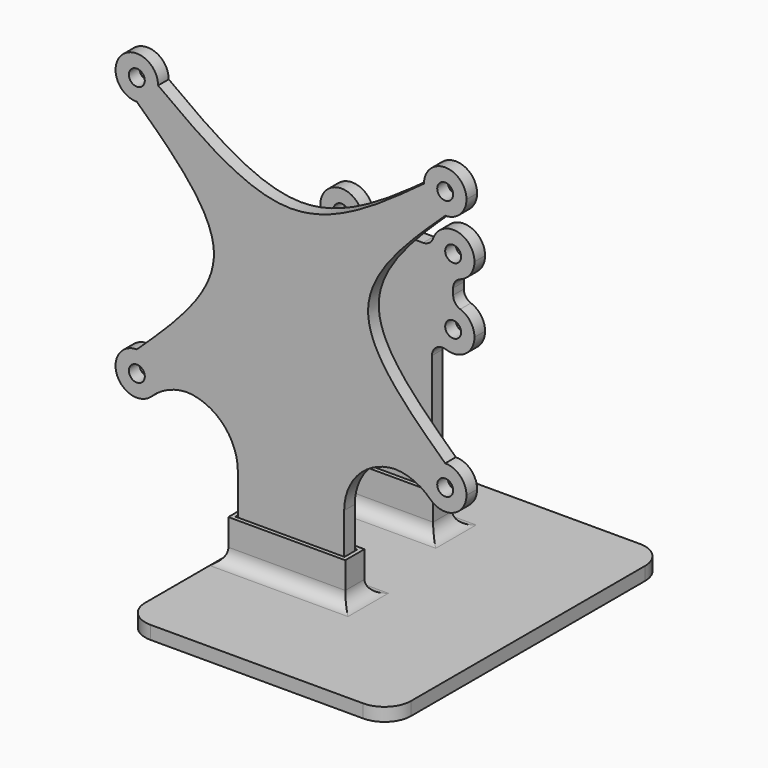
from build123d import *

# Parameters (mm, degrees)
F0_R          = 1.5
F1_DEPTH      = 2.5
F2_T1_DEPTH   = 2.5
F4_R          = 1.5
F4_W          = 13
F4_H          = 30
F5_DEPTH      = 2.5
F6_R          = 2
F7_R          = 2
F9_W          = 25
F9_H          = 65
F9_W_2        = 22
F9_H_2        = 4.5
F9_W_3        = 15
F9_W_4        = 20.5
F9_H_3        = 3
F9_W_5        = 13.5
F10_DEPTH     = 2.5
F11_DEPTH     = 7.5
F12_R         = 5
F13_T1_DEPTH  = 15
F13_T3_DEPTH  = 22
F13_T5_DEPTH  = 4.5
F13_T7_DEPTH  = 4.5
F13_T13_DEPTH = 10.75
F13_T17_DEPTH = 21.25
F13_T24_DEPTH = 21.25
F13_T29_DEPTH = 10.75
F13_T36_DEPTH = 10.75
F13_T40_DEPTH = 28.25
F13_T47_DEPTH = 28.25
F13_T52_DEPTH = 10.2282196187
F13_T59_DEPTH = 21.25
F13_T64_DEPTH = 10.75
F13_T71_DEPTH = 28.25
F13_T76_DEPTH = 10.2282196187
F13_T83_DEPTH = 21.25
F13_T87_DEPTH = 10.75
F13_T94_DEPTH = 28.25
F13_T98_DEPTH = 10.75


# Not quite as in the source:
# - a fillet or chamfer that OpenCascade refuses, or shapes differently, is made with other operations: its cross-section is extruded or revolved along the edge and cut away or added


with BuildPart() as f1:
    # F0 (on Front) → F1 (new body)
    with BuildSketch(Plane.XZ):
        with BuildLine():
            ThreePointArc((-29, 65), (-26.1715728753, 66.1715728753), (-25, 69))
            ThreePointArc((-25, 69), (-31.8284271247, 71.8284271247), (-29, 65))
        make_face()
        with Locations((-29, 69)):
            Circle(F0_R, mode=Mode.SUBTRACT)
        with BuildLine():
            add(Edge.make_bspline(
                [(-25, 69), (-16.6666666667, 62.875), (0, 50.625), (16.6666666667, 62.875), (25, 69)],
                knots=[0, 0, 0, 0, 0.5, 1, 1, 1, 1], degree=3))
            ThreePointArc((-25, 69), (-26.1715728753, 66.1715728753), (-29, 65))
            add(Edge.make_bspline(
                [(-29, 65), (-21.75, 58.1666666667), (-7.25, 44.5), (-21.75, 30.8333333333), (-29, 24)],
                knots=[0, 0, 0, 0, 0.5, 1, 1, 1, 1], degree=3))
            ThreePointArc((-29, 24), (-26.1715728753, 22.8284271247), (-25, 20))
            Line((-25, 20), (-10, 20))
            Line((-10, 20), (-10, 0))
            Line((-10, 0), (10, 0))
            Line((10, 0), (10, 20))
            Line((10, 20), (25, 20))
            ThreePointArc((25, 20), (26.1715728753, 22.8284271247), (29, 24))
            add(Edge.make_bspline(
                [(29, 65), (21.75, 58.1666666667), (7.25, 44.5), (21.75, 30.8333333333), (29, 24)],
                knots=[0, 0, 0, 0, 0.5, 1, 1, 1, 1], degree=3))
            ThreePointArc((29, 65), (26.1715728753, 66.1715728753), (25, 69))
        make_face()
        with BuildLine():
            ThreePointArc((33, 69), (29, 73), (25, 69))
            ThreePointArc((25, 69), (26.1715728753, 66.1715728753), (29, 65))
            ThreePointArc((29, 65), (31.8284271247, 66.1715728753), (33, 69))
        make_face()
        with Locations((29, 69)):
            Circle(F0_R, mode=Mode.SUBTRACT)
        with BuildLine():
            ThreePointArc((-25, 20), (-26.1715728753, 22.8284271247), (-29, 24))
            ThreePointArc((-29, 24), (-31.8284271247, 17.1715728753), (-25, 20))
        make_face()
        with Locations((-29, 20)):
            Circle(F0_R, mode=Mode.SUBTRACT)
        with BuildLine():
            ThreePointArc((33, 20), (31.8284271247, 22.8284271247), (29, 24))
            ThreePointArc((29, 24), (26.1715728753, 22.8284271247), (25, 20))
            ThreePointArc((25, 20), (29, 16), (33, 20))
        make_face()
        with Locations((29, 20)):
            Circle(F0_R, mode=Mode.SUBTRACT)
    extrude(amount=F1_DEPTH)

    # F2: fillet of radius 10 on 4 edges, made by hand

    # F2_s2 → F2_t1 (join)
    with BuildSketch(Plane.XZ):
        with BuildLine():
            ThreePointArc((-26.2005831511, 17.1428571429), (-22.981685759, 19.2582009977), (-19.2020410289, 20))
            Line((-19.2020410289, 20), (-25, 20))
            ThreePointArc((-25, 20), (-25.3123403495, 18.4504302848), (-26.2005831511, 17.1428571429))
        make_face()
        with BuildLine():
            ThreePointArc((19.2020410289, 20), (22.981685759, 19.2582009977), (26.2005831511, 17.1428571429))
            ThreePointArc((26.2005831511, 17.1428571429), (25.3123403495, 18.4504302848), (25, 20))
            Line((25, 20), (19.2020410289, 20))
        make_face()
        with BuildLine():
            ThreePointArc((-20, 20), (-12.9289321881, 17.0710678119), (-10, 10))
            Line((-10, 10), (-10, 20))
            Line((-10, 20), (-20, 20))
        make_face()
        with BuildLine():
            ThreePointArc((10, 10), (12.9289321881, 17.0710678119), (20, 20))
            Line((20, 20), (10, 20))
            Line((10, 20), (10, 10))
        make_face()
    extrude(amount=F2_T1_DEPTH)


with BuildPart() as f5:
    # F4 (on offset) → F5 (new body)
    with BuildSketch(Plane.XZ.offset(-25)):
        with BuildLine():
            ThreePointArc((-10.5, 38.5), (-7.6715728753, 39.6715728753), (-6.5, 42.5))
            ThreePointArc((-6.5, 42.5), (-13.3284271247, 45.3284271247), (-10.5, 38.5))
        make_face()
        with Locations((-10.5, 42.5)):
            Circle(F4_R, mode=Mode.SUBTRACT)
        with BuildLine():
            Line((6.5, 42.5), (-6.5, 42.5))
            ThreePointArc((-6.5, 42.5), (-7.6715728753, 39.6715728753), (-10.5, 38.5))
            Line((-10.5, 38.5), (-10.5, 34))
            ThreePointArc((-10.5, 34), (-7.6715728753, 32.8284271247), (-6.5, 30))
            Line((-6.5, 30), (6.5, 30))
            ThreePointArc((6.5, 30), (7.6715728753, 32.8284271247), (10.5, 34))
            Line((10.5, 34), (10.5, 38.5))
            ThreePointArc((10.5, 38.5), (7.6715728753, 39.6715728753), (6.5, 42.5))
        make_face()
        with BuildLine():
            ThreePointArc((14.5, 42.5), (10.5, 46.5), (6.5, 42.5))
            ThreePointArc((6.5, 42.5), (7.6715728753, 39.6715728753), (10.5, 38.5))
            ThreePointArc((10.5, 38.5), (13.3284271247, 39.6715728753), (14.5, 42.5))
        make_face()
        with Locations((10.5, 42.5)):
            Circle(F4_R, mode=Mode.SUBTRACT)
        with BuildLine():
            ThreePointArc((-6.5, 30), (-7.6715728753, 32.8284271247), (-10.5, 34))
            ThreePointArc((-10.5, 34), (-13.3284271247, 27.1715728753), (-6.5, 30))
        make_face()
        with Locations((-10.5, 30)):
            Circle(F4_R, mode=Mode.SUBTRACT)
        with Locations((0, 15)):
            Rectangle(F4_W, F4_H)
        with BuildLine():
            ThreePointArc((14.5, 30), (13.3284271247, 32.8284271247), (10.5, 34))
            ThreePointArc((10.5, 34), (7.6715728753, 32.8284271247), (6.5, 30))
            ThreePointArc((6.5, 30), (10.5, 26), (14.5, 30))
        make_face()
        with Locations((10.5, 30)):
            Circle(F4_R, mode=Mode.SUBTRACT)
    extrude(amount=F5_DEPTH)

    # F6
    f6_edges = [f5.edges().sort_by_distance(p)[0] for p in [
        (-6.5, 23.75, 42.5),
        (6.5, 23.75, 42.5),
        (10.5, 23.75, 38.5),
        (-10.5, 23.75, 38.5),
        (-10.5, 23.75, 34),
        (10.5, 23.75, 34),
    ]]
    fillet(f6_edges, radius=F6_R)

    # F7
    f7_edges = [f5.edges().sort_by_distance(p)[0] for p in [
        (-6.5, 23.75, 30),
        (6.5, 23.75, 30),
    ]]
    fillet(f7_edges, radius=F7_R)


with BuildPart() as f10:
    # F9 (on offset) → F10 (new body)
    with BuildSketch(Plane.XY.offset(-5)):
        with Locations((0, 6.3541418326)):
            Rectangle(F9_W, F9_H)
        with Locations((0, -1.238761819)):
            Rectangle(F9_W_2, F9_H_2, mode=Mode.SUBTRACT)
        with Locations((0, 23.7820465118)):
            Rectangle(F9_W_3, F9_H_2, mode=Mode.SUBTRACT)
        with Locations((25, 6.3541418326)):
            Rectangle(F9_W, F9_H)
        with Locations((0, -1.238761819)):
            Rectangle(F9_W_2, F9_H_2)
        with Locations((0, -1.238761819)):
            Rectangle(F9_W_4, F9_H_3, mode=Mode.SUBTRACT)
        with Locations((0, 23.7820465118)):
            Rectangle(F9_W_3, F9_H_2)
        with Locations((0, 23.7820465118)):
            Rectangle(F9_W_5, F9_H_3, mode=Mode.SUBTRACT)
        with Locations((0, -1.238761819)):
            Rectangle(F9_W_4, F9_H_3)
        with Locations((0, 23.7820465118)):
            Rectangle(F9_W_5, F9_H_3)
    extrude(amount=-F10_DEPTH)

    # F9 (on offset) → F11 (join)
    with BuildSketch(Plane.XY.offset(-5)):
        with Locations((0, 23.7820465118)):
            Rectangle(F9_W_3, F9_H_2)
        with Locations((0, 23.7820465118)):
            Rectangle(F9_W_5, F9_H_3, mode=Mode.SUBTRACT)
        with Locations((0, -1.238761819)):
            Rectangle(F9_W_2, F9_H_2)
        with Locations((0, -1.238761819)):
            Rectangle(F9_W_4, F9_H_3, mode=Mode.SUBTRACT)
    extrude(amount=F11_DEPTH)

    # F12
    f12_edges = [f10.edges().sort_by_distance(p)[0] for p in [
        (-12.5, 38.854142, -6.25),
        (-12.5, -26.145858, -6.25),
        (37.5, -26.145858, -6.25),
        (37.5, 38.854142, -6.25),
    ]]
    fillet(f12_edges, radius=F12_R)

    # F13: fillet of radius 2.5 on 8 edges, made by hand

    # F13_s2 → F13_t1 (join)
    with BuildSketch(Plane.YZ.offset(-7.5)):
        with BuildLine():
            ThreePointArc((28.5320465118, -5), (26.7642795588, -4.267766953), (26.0320465118, -2.5))
            Line((26.0320465118, -2.5), (26.0320465118, -5))
            Line((26.0320465118, -5), (28.5320465118, -5))
        make_face()
        with BuildLine():
            ThreePointArc((19.0320465118, -5), (20.7998134647, -4.267766953), (21.5320465118, -2.5))
            Line((21.5320465118, -2.5), (21.5320465118, -5))
            Line((21.5320465118, -5), (19.0320465118, -5))
        make_face()
    extrude(amount=F13_T1_DEPTH)

    # F13_s4 → F13_t3 (join)
    with BuildSketch(Plane.YZ.offset(-11)):
        with BuildLine():
            ThreePointArc((3.511238181, -5), (1.7434712281, -4.267766953), (1.011238181, -2.5))
            Line((1.011238181, -2.5), (1.011238181, -5))
            Line((1.011238181, -5), (3.511238181, -5))
        make_face()
        with BuildLine():
            ThreePointArc((-5.988761819, -5), (-4.220994866, -4.267766953), (-3.488761819, -2.5))
            Line((-3.488761819, -2.5), (-3.488761819, -5))
            Line((-3.488761819, -5), (-5.988761819, -5))
        make_face()
    extrude(amount=F13_T3_DEPTH)

    # F13_s6 → F13_t5 (join)
    with BuildSketch(Plane.XZ.offset(-26.0320465118)):
        with BuildLine():
            ThreePointArc((-10, -5), (-8.232233047, -4.267766953), (-7.5, -2.5))
            Line((-7.5, -2.5), (-7.5, -5))
            Line((-7.5, -5), (-10, -5))
        make_face()
        with BuildLine():
            ThreePointArc((10, -5), (8.232233047, -4.267766953), (7.5, -2.5))
            Line((7.5, -2.5), (7.5, -5))
            Line((7.5, -5), (10, -5))
        make_face()
    extrude(amount=F13_T5_DEPTH)

    # F13_s8 → F13_t7 (join)
    with BuildSketch(Plane.XZ.offset(-1.011238181)):
        with BuildLine():
            ThreePointArc((-12.5, -5), (-11.4083499337, -4.0780185463), (-11, -2.7087121525))
            Line((-11, -2.7087121525), (-11, -5))
            Line((-11, -5), (-12.5, -5))
        make_face()
        with BuildLine():
            ThreePointArc((13.5, -5), (11.732233047, -4.267766953), (11, -2.5))
            Line((11, -2.5), (11, -5))
            Line((11, -5), (13.5, -5))
        make_face()
    extrude(amount=F13_T7_DEPTH)


with BuildPart() as f13_tool11:
    # F13_s12 → F13_t13 (new body)
    with BuildSketch(Plane.XZ.offset(-21.5320465118)):
        with BuildLine():
            ThreePointArc((10, -5), (8.232233047, -4.267766953), (7.5, -2.5))
            Line((7.5, -2.5), (7.5, -5))
            Line((7.5, -5), (10, -5))
        make_face()
    extrude(amount=-F13_T13_DEPTH)

    split(bisect_by=Plane.XZ.offset(-26.0320465118), keep=Keep.BOTTOM)


with BuildPart() as f13_tool15:
    # F13_s16 → F13_t17 (new body)
    with BuildSketch(Plane.YZ.offset(13.75)):
        with BuildLine():
            ThreePointArc((28.5320465118, -5), (26.7642795588, -4.267766953), (26.0320465118, -2.5))
            Line((26.0320465118, -2.5), (26.0320465118, -5))
            Line((26.0320465118, -5), (28.5320465118, -5))
        make_face()
    extrude(amount=-F13_T17_DEPTH)

    split(bisect_by=Plane.YZ.offset(7.5), keep=Keep.TOP)


with BuildPart() as f13_tool11_1:
    add(f13_tool11.part)

    # F13_t19: intersect F13_tool15
    add(f13_tool15.part, mode=Mode.INTERSECT)


with BuildPart() as f10_1:
    add(f10.part)

    # F13_t9: union F13_tool11
    add(f13_tool11_1.part)


with BuildPart() as f13_tool22:
    # F13_s23 → F13_t24 (new body)
    with BuildSketch(Plane.YZ.offset(7.5)):
        with BuildLine():
            ThreePointArc((28.5320465118, -5), (26.7642795588, -4.267766953), (26.0320465118, -2.5))
            Line((26.0320465118, -2.5), (26.0320465118, -5))
            Line((26.0320465118, -5), (28.5320465118, -5))
        make_face()
    extrude(amount=-F13_T24_DEPTH)

    split(bisect_by=Plane.YZ.offset(-12.5), keep=Keep.TOP)

    split(bisect_by=Plane.YZ.offset(-7.5), keep=Keep.BOTTOM)


with BuildPart() as f13_tool27:
    # F13_s28 → F13_t29 (new body)
    with BuildSketch(Plane.XZ.offset(-32.2820465118)):
        with BuildLine():
            ThreePointArc((-10, -5), (-8.232233047, -4.267766953), (-7.5, -2.5))
            Line((-7.5, -2.5), (-7.5, -5))
            Line((-7.5, -5), (-10, -5))
        make_face()
    extrude(amount=F13_T29_DEPTH)

    split(bisect_by=Plane.XZ.offset(-26.0320465118), keep=Keep.BOTTOM)


with BuildPart() as f13_tool22_1:
    add(f13_tool22.part)

    # F13_t31: intersect F13_tool27
    add(f13_tool27.part, mode=Mode.INTERSECT)


with BuildPart() as f10_2:
    add(f10_1.part)

    # F13_t20: union F13_tool22
    add(f13_tool22_1.part)


with BuildPart() as f13_tool34:
    # F13_s35 → F13_t36 (new body)
    with BuildSketch(Plane.XZ.offset(3.488761819)):
        with BuildLine():
            ThreePointArc((13.5, -5), (11.732233047, -4.267766953), (11, -2.5))
            Line((11, -2.5), (11, -5))
            Line((11, -5), (13.5, -5))
        make_face()
    extrude(amount=-F13_T36_DEPTH)

    split(bisect_by=Plane.XZ.offset(-1.011238181), keep=Keep.BOTTOM)


with BuildPart() as f13_tool38:
    # F13_s39 → F13_t40 (new body)
    with BuildSketch(Plane.YZ.offset(17.25)):
        with BuildLine():
            ThreePointArc((3.511238181, -5), (1.7434712281, -4.267766953), (1.011238181, -2.5))
            Line((1.011238181, -2.5), (1.011238181, -5))
            Line((1.011238181, -5), (3.511238181, -5))
        make_face()
    extrude(amount=-F13_T40_DEPTH)

    split(bisect_by=Plane.YZ.offset(11), keep=Keep.TOP)


with BuildPart() as f13_tool34_1:
    add(f13_tool34.part)

    # F13_t42: intersect F13_tool38
    add(f13_tool38.part, mode=Mode.INTERSECT)


with BuildPart() as f10_3:
    add(f10_2.part)

    # F13_t32: union F13_tool34
    add(f13_tool34_1.part)


with BuildPart() as f13_tool45:
    # F13_s46 → F13_t47 (new body)
    with BuildSketch(Plane.YZ.offset(11)):
        with BuildLine():
            ThreePointArc((3.511238181, -5), (1.7434712281, -4.267766953), (1.011238181, -2.5))
            Line((1.011238181, -2.5), (1.011238181, -5))
            Line((1.011238181, -5), (3.511238181, -5))
        make_face()
    extrude(amount=-F13_T47_DEPTH)

    split(bisect_by=Plane.YZ.offset(-12.5), keep=Keep.TOP)

    split(bisect_by=Plane.YZ.offset(-11), keep=Keep.BOTTOM)


with BuildPart() as f13_tool50:
    # F13_s51 → F13_t52 (new body)
    with BuildSketch(Plane.XZ.offset(-6.7394577997)):
        with BuildLine():
            ThreePointArc((-12.5, -5), (-11.4083499337, -4.0780185463), (-11, -2.7087121525))
            Line((-11, -2.7087121525), (-11, -5))
            Line((-11, -5), (-12.5, -5))
        make_face()
    extrude(amount=F13_T52_DEPTH)

    split(bisect_by=Plane.XZ.offset(-1.011238181), keep=Keep.BOTTOM)


with BuildPart() as f13_tool45_1:
    add(f13_tool45.part)

    # F13_t54: intersect F13_tool50
    add(f13_tool50.part, mode=Mode.INTERSECT)


with BuildPart() as f10_4:
    add(f10_3.part)

    # F13_t43: union F13_tool45
    add(f13_tool45_1.part)


with BuildPart() as f13_tool57:
    # F13_s58 → F13_t59 (new body)
    with BuildSketch(Plane.YZ.offset(-13.75)):
        with BuildLine():
            ThreePointArc((19.0320465118, -5), (20.7998134647, -4.267766953), (21.5320465118, -2.5))
            Line((21.5320465118, -2.5), (21.5320465118, -5))
            Line((21.5320465118, -5), (19.0320465118, -5))
        make_face()
    extrude(amount=F13_T59_DEPTH)

    split(bisect_by=Plane.YZ.offset(-12.5), keep=Keep.TOP)

    split(bisect_by=Plane.YZ.offset(-7.5), keep=Keep.BOTTOM)


with BuildPart() as f13_tool62:
    # F13_s63 → F13_t64 (new body)
    with BuildSketch(Plane.XZ.offset(-26.0320465118)):
        with BuildLine():
            ThreePointArc((-10, -5), (-8.232233047, -4.267766953), (-7.5, -2.5))
            Line((-7.5, -2.5), (-7.5, -5))
            Line((-7.5, -5), (-10, -5))
        make_face()
    extrude(amount=F13_T64_DEPTH)

    split(bisect_by=Plane.XZ.offset(-21.5320465118), keep=Keep.TOP)


with BuildPart() as f13_tool57_1:
    add(f13_tool57.part)

    # F13_t66: intersect F13_tool62
    add(f13_tool62.part, mode=Mode.INTERSECT)


with BuildPart() as f10_5:
    add(f10_4.part)

    # F13_t55: union F13_tool57
    add(f13_tool57_1.part)


with BuildPart() as f13_tool69:
    # F13_s70 → F13_t71 (new body)
    with BuildSketch(Plane.YZ.offset(-17.25)):
        with BuildLine():
            ThreePointArc((-5.988761819, -5), (-4.220994866, -4.267766953), (-3.488761819, -2.5))
            Line((-3.488761819, -2.5), (-3.488761819, -5))
            Line((-3.488761819, -5), (-5.988761819, -5))
        make_face()
    extrude(amount=F13_T71_DEPTH)

    split(bisect_by=Plane.YZ.offset(-12.5), keep=Keep.TOP)

    split(bisect_by=Plane.YZ.offset(-11), keep=Keep.BOTTOM)


with BuildPart() as f13_tool74:
    # F13_s75 → F13_t76 (new body)
    with BuildSketch(Plane.XZ.offset(-1.011238181)):
        with BuildLine():
            ThreePointArc((-12.5, -5), (-11.4083499337, -4.0780185463), (-11, -2.7087121525))
            Line((-11, -2.7087121525), (-11, -5))
            Line((-11, -5), (-12.5, -5))
        make_face()
    extrude(amount=F13_T76_DEPTH)

    split(bisect_by=Plane.XZ.offset(3.488761819), keep=Keep.TOP)


with BuildPart() as f13_tool69_1:
    add(f13_tool69.part)

    # F13_t78: intersect F13_tool74
    add(f13_tool74.part, mode=Mode.INTERSECT)


with BuildPart() as f10_6:
    add(f10_5.part)

    # F13_t67: union F13_tool69
    add(f13_tool69_1.part)


with BuildPart() as f13_tool81:
    # F13_s82 → F13_t83 (new body)
    with BuildSketch(Plane.YZ.offset(-7.5)):
        with BuildLine():
            ThreePointArc((19.0320465118, -5), (20.7998134647, -4.267766953), (21.5320465118, -2.5))
            Line((21.5320465118, -2.5), (21.5320465118, -5))
            Line((21.5320465118, -5), (19.0320465118, -5))
        make_face()
    extrude(amount=F13_T83_DEPTH)

    split(bisect_by=Plane.YZ.offset(7.5), keep=Keep.TOP)


with BuildPart() as f13_tool85:
    # F13_s86 → F13_t87 (new body)
    with BuildSketch(Plane.XZ.offset(-15.2820465118)):
        with BuildLine():
            ThreePointArc((10, -5), (8.232233047, -4.267766953), (7.5, -2.5))
            Line((7.5, -2.5), (7.5, -5))
            Line((7.5, -5), (10, -5))
        make_face()
    extrude(amount=-F13_T87_DEPTH)

    split(bisect_by=Plane.XZ.offset(-21.5320465118), keep=Keep.TOP)


with BuildPart() as f13_tool81_1:
    add(f13_tool81.part)

    # F13_t89: intersect F13_tool85
    add(f13_tool85.part, mode=Mode.INTERSECT)


with BuildPart() as f10_7:
    add(f10_6.part)

    # F13_t79: union F13_tool81
    add(f13_tool81_1.part)


with BuildPart() as f13_tool92:
    # F13_s93 → F13_t94 (new body)
    with BuildSketch(Plane.YZ.offset(-11)):
        with BuildLine():
            ThreePointArc((-5.988761819, -5), (-4.220994866, -4.267766953), (-3.488761819, -2.5))
            Line((-3.488761819, -2.5), (-3.488761819, -5))
            Line((-3.488761819, -5), (-5.988761819, -5))
        make_face()
    extrude(amount=F13_T94_DEPTH)

    split(bisect_by=Plane.YZ.offset(11), keep=Keep.TOP)


with BuildPart() as f13_tool96:
    # F13_s97 → F13_t98 (new body)
    with BuildSketch(Plane.XZ.offset(9.738761819)):
        with BuildLine():
            ThreePointArc((13.5, -5), (11.732233047, -4.267766953), (11, -2.5))
            Line((11, -2.5), (11, -5))
            Line((11, -5), (13.5, -5))
        make_face()
    extrude(amount=-F13_T98_DEPTH)

    split(bisect_by=Plane.XZ.offset(3.488761819), keep=Keep.TOP)


with BuildPart() as f13_tool92_1:
    add(f13_tool92.part)

    # F13_t100: intersect F13_tool96
    add(f13_tool96.part, mode=Mode.INTERSECT)


with BuildPart() as f10_8:
    add(f10_7.part)

    # F13_t90: union F13_tool92
    add(f13_tool92_1.part)


solid = Compound([f1.part, f5.part, f10_8.part])
